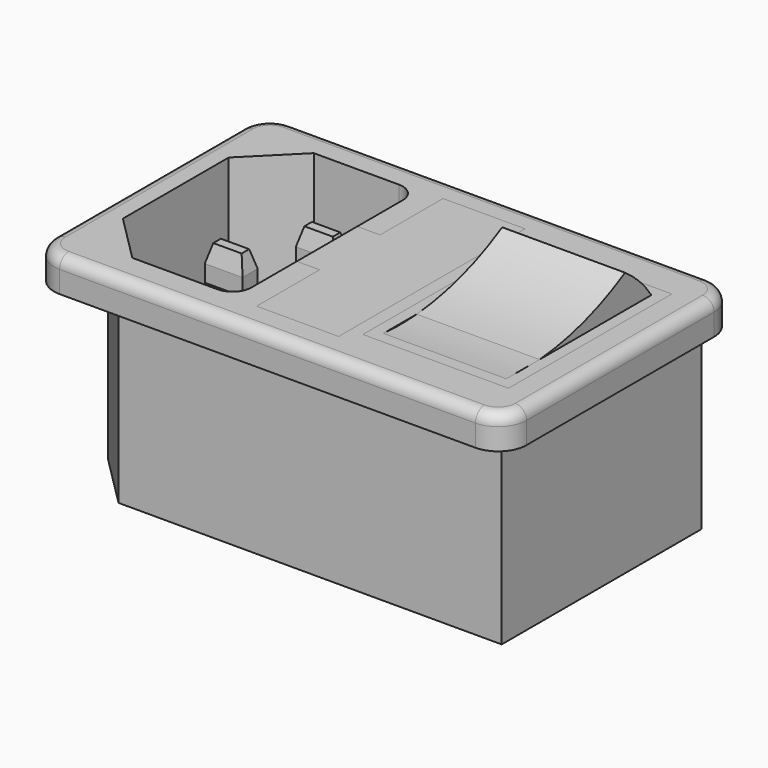
from build123d import *

# Parameters (mm, degrees)
F0_W        = 15.4
F0_H        = 21.6
F1_DEPTH    = 3.5
F0_W_2      = 4
F0_H_2      = 2
F0_W_3      = 13
F0_H_3      = 19.2
F0_W_4      = 2.418700546
F0_H_4      = 8
F2_DEPTH    = 19
F3_DEPTH    = 15
F4_C1_SIZE2 = 0.5
F4_C1_SIZE  = 1.8660254038
F4_C2_SIZE2 = 0.5
F4_C2_SIZE  = 1.8660254038
F4_C3_SIZE2 = 1.8660254038
F4_C3_SIZE  = 0.5
F4_C4_SIZE2 = 1.8660254038
F4_C4_SIZE  = 0.5
F5_SIZE2    = 1.8660254038
F5_SIZE     = 0.5
F6_SIZE2    = 1.8660254038
F6_SIZE     = 0.5
F7_DEPTH    = 3.5
F8_DEPTH    = 22
F10_DEPTH   = 25
F11_R       = 1.2
F12_START   = -14.9
F12_DEPTH   = 0.1


with BuildPart() as f1:
    # F0 (on Top) → F1 (new body)
    with BuildSketch(Plane.XY):
        with BuildLine():
            Line((21.4106866419, 15.232257545), (-22.5893133581, 15.232257545))
            ThreePointArc((-22.5893133581, 15.232257545), (-24.7106337016, 14.3535778886), (-25.5893133581, 12.232257545))
            Line((-25.5893133581, 12.232257545), (-25.5893133581, -12.567742455))
            ThreePointArc((-25.5893133581, -12.567742455), (-24.7106337016, -14.6890627986), (-22.5893133581, -15.567742455))
            Line((-22.5893133581, -15.567742455), (21.4106866419, -15.567742455))
            ThreePointArc((21.4106866419, -15.567742455), (23.5320069855, -14.6890627986), (24.4106866419, -12.567742455))
            Line((24.4106866419, -12.567742455), (24.4106866419, 12.232257545))
            ThreePointArc((24.4106866419, 12.232257545), (23.5320069855, 14.3535778886), (21.4106866419, 15.232257545))
        make_face()
        Polygon((-18.2525572471, 13.2), (-8.7555009723, 13.2), (22.2888856925, 13.2), (22.2888856925, -13.2), (-8.7555009723, -13.2), (-18.2525572471, -13.2), (-23.9555009723, -7.4970562748), (-23.9555009723, 7.4970562748), align=None, mode=Mode.SUBTRACT)
        Polygon((22.2888856925, 13.2), (-8.7555009723, 13.2), (-18.2525572471, 13.2), (-23.9555009723, 7.4970562748), (-23.9555009723, -7.4970562748), (-18.2525572471, -13.2), (-8.7555009723, -13.2), (22.2888856925, -13.2), align=None)
        with BuildLine():
            Line((-4.3368004262, 4), (-4.3368004262, 12.3322419822))
            Line((-4.3368004262, 12.3322419822), (4.3368004262, 12.3322419822))
            Line((4.3368004262, 12.3322419822), (4.3368004262, -12.3322419822))
            Line((4.3368004262, -12.3322419822), (-4.3368004262, -12.3322419822))
            Line((-4.3368004262, -12.3322419822), (-4.3368004262, -4))
            Line((-4.3368004262, -4), (-6.7555009723, -4))
            Line((-6.7555009723, -4), (-6.7555009723, -10))
            ThreePointArc((-6.7555009723, -10), (-7.3412874099, -11.4142135624), (-8.7555009723, -12))
            Line((-8.7555009723, -12), (-17.7555009723, -12))
            Line((-17.7555009723, -12), (-22.7555009723, -7))
            Line((-22.7555009723, -7), (-22.7555009723, 7))
            Line((-22.7555009723, 7), (-17.7555009723, 12))
            Line((-17.7555009723, 12), (-8.7555009723, 12))
            ThreePointArc((-8.7555009723, 12), (-7.3412874099, 11.4142135624), (-6.7555009723, 10))
            Line((-6.7555009723, 10), (-6.7555009723, 4))
            Line((-6.7555009723, 4), (-4.3368004262, 4))
        make_face(mode=Mode.SUBTRACT)
        with Locations((13.3888856925, 0)):
            Rectangle(F0_W, F0_H, mode=Mode.SUBTRACT)
    extrude(amount=F1_DEPTH)

    # F0 (on Top) → F2 (join)
    with BuildSketch(Plane.XY):
        Polygon((22.2888856925, 13.2), (-8.7555009723, 13.2), (-18.2525572471, 13.2), (-23.9555009723, 7.4970562748), (-23.9555009723, -7.4970562748), (-18.2525572471, -13.2), (-8.7555009723, -13.2), (22.2888856925, -13.2), align=None)
        with BuildLine():
            Line((-4.3368004262, 4), (-4.3368004262, 12.3322419822))
            Line((-4.3368004262, 12.3322419822), (4.3368004262, 12.3322419822))
            Line((4.3368004262, 12.3322419822), (4.3368004262, -12.3322419822))
            Line((4.3368004262, -12.3322419822), (-4.3368004262, -12.3322419822))
            Line((-4.3368004262, -12.3322419822), (-4.3368004262, -4))
            Line((-4.3368004262, -4), (-6.7555009723, -4))
            Line((-6.7555009723, -4), (-6.7555009723, -10))
            ThreePointArc((-6.7555009723, -10), (-7.3412874099, -11.4142135624), (-8.7555009723, -12))
            Line((-8.7555009723, -12), (-17.7555009723, -12))
            Line((-17.7555009723, -12), (-22.7555009723, -7))
            Line((-22.7555009723, -7), (-22.7555009723, 7))
            Line((-22.7555009723, 7), (-17.7555009723, 12))
            Line((-17.7555009723, 12), (-8.7555009723, 12))
            ThreePointArc((-8.7555009723, 12), (-7.3412874099, 11.4142135624), (-6.7555009723, 10))
            Line((-6.7555009723, 10), (-6.7555009723, 4))
            Line((-6.7555009723, 4), (-4.3368004262, 4))
        make_face(mode=Mode.SUBTRACT)
        with Locations((13.3888856925, 0)):
            Rectangle(F0_W, F0_H, mode=Mode.SUBTRACT)
        with BuildLine():
            Line((-6.7555009723, -4), (-6.7555009723, 4))
            Line((-6.7555009723, 4), (-6.7555009723, 10))
            ThreePointArc((-6.7555009723, 10), (-7.3412874099, 11.4142135624), (-8.7555009723, 12))
            Line((-8.7555009723, 12), (-17.7555009723, 12))
            Line((-17.7555009723, 12), (-22.7555009723, 7))
            Line((-22.7555009723, 7), (-22.7555009723, -7))
            Line((-22.7555009723, -7), (-17.7555009723, -12))
            Line((-17.7555009723, -12), (-8.7555009723, -12))
            ThreePointArc((-8.7555009723, -12), (-7.3412874099, -11.4142135624), (-6.7555009723, -10))
            Line((-6.7555009723, -10), (-6.7555009723, -4))
        make_face()
        with Locations((-12.8875139207, -6.9733052514)):
            Rectangle(F0_W_2, F0_H_2, mode=Mode.SUBTRACT)
        with Locations((-16.8875139207, 0)):
            Rectangle(F0_W_2, F0_H_2, mode=Mode.SUBTRACT)
        with Locations((-12.8875139207, 7.0500936662)):
            Rectangle(F0_W_2, F0_H_2, mode=Mode.SUBTRACT)
        with Locations((13.3888856925, 0)):
            Rectangle(F0_W, F0_H)
        with Locations((13.3888856925, 0)):
            Rectangle(F0_W_3, F0_H_3, mode=Mode.SUBTRACT)
        with Locations((13.3888856925, 0)):
            Rectangle(F0_W_3, F0_H_3)
        Polygon((4.3368004262, 12.3322419822), (-4.3368004262, 12.3322419822), (-4.3368004262, 4), (-4.3368004262, -4), (-4.3368004262, -12.3322419822), (4.3368004262, -12.3322419822), align=None)
        with Locations((-5.5461506993, 0)):
            Rectangle(F0_W_4, F0_H_4)
        with Locations((-12.8875139207, -6.9733052514)):
            Rectangle(F0_W_2, F0_H_2)
        with Locations((-16.8875139207, 0)):
            Rectangle(F0_W_2, F0_H_2)
        with Locations((-12.8875139207, 7.0500936662)):
            Rectangle(F0_W_2, F0_H_2)
    extrude(amount=-F2_DEPTH)

    # F0 (on Top) → F3 (cut)
    with BuildSketch(Plane.XY):
        with BuildLine():
            Line((-6.7555009723, -4), (-6.7555009723, 4))
            Line((-6.7555009723, 4), (-6.7555009723, 10))
            ThreePointArc((-6.7555009723, 10), (-7.3412874099, 11.4142135624), (-8.7555009723, 12))
            Line((-8.7555009723, 12), (-17.7555009723, 12))
            Line((-17.7555009723, 12), (-22.7555009723, 7))
            Line((-22.7555009723, 7), (-22.7555009723, -7))
            Line((-22.7555009723, -7), (-17.7555009723, -12))
            Line((-17.7555009723, -12), (-8.7555009723, -12))
            ThreePointArc((-8.7555009723, -12), (-7.3412874099, -11.4142135624), (-6.7555009723, -10))
            Line((-6.7555009723, -10), (-6.7555009723, -4))
        make_face()
        with Locations((-12.8875139207, -6.9733052514)):
            Rectangle(F0_W_2, F0_H_2, mode=Mode.SUBTRACT)
        with Locations((-16.8875139207, 0)):
            Rectangle(F0_W_2, F0_H_2, mode=Mode.SUBTRACT)
        with Locations((-12.8875139207, 7.0500936662)):
            Rectangle(F0_W_2, F0_H_2, mode=Mode.SUBTRACT)
        with Locations((13.3888856925, 0)):
            Rectangle(F0_W_3, F0_H_3)
    extrude(amount=-F3_DEPTH, mode=Mode.SUBTRACT)

    # F4: chamfer of 0.5 x 1.8660254038 on 4 edges, made by hand

    # F4_c1
    f4_c1_edges = [f1.edges().sort_by_distance(p)[0] for p in [
        (-10.8875139207, 7.0500936662, 0),
    ]]
    f4_c1_side = f1.faces().sort_by_distance((-10.8875139207, 7.0500936662, -0.01))[0]
    chamfer(f4_c1_edges, length=F4_C1_SIZE, length2=F4_C1_SIZE2, reference=f4_c1_side)

    # F4_c2
    f4_c2_edges = [f1.edges().sort_by_distance(p)[0] for p in [
        (-13.1375139207, 6.0500936662, 0),
    ]]
    f4_c2_side = f1.faces().sort_by_distance((-13.1375139207, 6.0500936662, -0.01))[0]
    chamfer(f4_c2_edges, length=F4_C2_SIZE, length2=F4_C2_SIZE2, reference=f4_c2_side)

    # F4_c3
    f4_c3_edges = [f1.edges().sort_by_distance(p)[0] for p in [
        (-14.8875139207, 7.3000936662, 0),
    ]]
    f4_c3_side = f1.faces().sort_by_distance((-14.8775139207, 7.3000936662, 0))[0]
    chamfer(f4_c3_edges, length=F4_C3_SIZE, length2=F4_C3_SIZE2, reference=f4_c3_side)

    # F4_c4
    f4_c4_edges = [f1.edges().sort_by_distance(p)[0] for p in [
        (-12.8875139207, 8.0500936662, 0),
    ]]
    f4_c4_side = f1.faces().sort_by_distance((-12.8875139207, 8.0400936662, 0))[0]
    chamfer(f4_c4_edges, length=F4_C4_SIZE, length2=F4_C4_SIZE2, reference=f4_c4_side)

    # F5
    f5_edges = [f1.edges().sort_by_distance(p)[0] for p in [
        (-16.887514, 1, 0),
        (-14.887514, 0, 0),
        (-16.887514, -1, 0),
        (-18.887514, 0, 0),
    ]]
    f5_side = f1.faces().sort_by_distance((-16.887514, 0, 0))[0]
    chamfer(f5_edges, length=F5_SIZE, length2=F5_SIZE2, reference=f5_side)

    # F6
    f6_edges = [f1.edges().sort_by_distance(p)[0] for p in [
        (-14.887514, -6.973305, 0),
        (-12.887514, -5.973305, 0),
        (-10.887514, -6.973305, 0),
        (-12.887514, -7.973305, 0),
    ]]
    f6_side = f1.faces().sort_by_distance((-12.887514, -6.973305, 0))[0]
    chamfer(f6_edges, length=F6_SIZE, length2=F6_SIZE2, reference=f6_side)


with BuildPart() as f7:
    # F7 (new, through all): a face of the model
    f7_faces = [f1.part.faces().sort_by_distance(p)[0] for p in [
        (-0.4600310991, 0, 0),
    ]]
    extrude(f7_faces, amount=F7_DEPTH)


with BuildPart() as f7b:
    # F7#2 (new, through all): a face of the model
    f7_2_faces = [f1.part.faces().sort_by_distance(p)[0] for p in [
        (13.3888856925, -10.5347227865, 0),
    ]]
    extrude(f7_2_faces, amount=F7_DEPTH)


with BuildPart() as f8:
    # F8 (new): a face of the model
    f8_faces = [f1.part.faces().sort_by_distance(p)[0] for p in [
        (13.3888856925, 0, -15),
    ]]
    extrude(f8_faces, amount=F8_DEPTH)

    # F9 (on face) → F10 (cut)
    with BuildSketch(Plane.YZ.offset(19.8888856925)):
        with BuildLine():
            ThreePointArc((-9.6, 3.5), (-7.3938840069, 3.410434439), (-5.1877680138, 3.5))
            Line((-5.1877680138, 3.5), (-9.6, 3.5))
        make_face()
        with BuildLine():
            Line((-9.6, 3.5), (-5.1877680138, 3.5))
            ThreePointArc((-5.1877680138, 3.5), (0.6561669902, 4.6282852574), (6.1150655176, 7))
            Line((6.1150655176, 7), (-9.6, 7))
            Line((-9.6, 7), (-9.6, 3.5))
        make_face()
        with BuildLine():
            ThreePointArc((6.1150655176, 7), (8.0179372576, 5.4097140483), (9.6, 3.5))
            Line((9.6, 3.5), (9.6, 7))
            Line((9.6, 7), (6.1150655176, 7))
        make_face()
    extrude(amount=-F10_DEPTH, mode=Mode.SUBTRACT)


with BuildPart() as f1_1:
    add(f1.part)

    # F11
    f11_edges = [f1_1.edges().sort_by_distance(p)[0] for p in [
        (-25.589313, -0.167742, 3.5),
        (24.410687, -0.167742, 3.5),
        (23.532007, 14.353578, 3.5),
        (-0.589313, 15.232258, 3.5),
        (-24.710634, 14.353578, 3.5),
        (-24.710634, -14.689063, 3.5),
        (-0.589313, -15.567742, 3.5),
        (23.532007, -14.689063, 3.5),
    ]]
    fillet(f11_edges, radius=F11_R)

    # F0 (on Top) → F12 (cut)
    with BuildSketch(Plane.XY.offset(F12_START)):
        with Locations((-12.8875139207, 7.0500936662)):
            Rectangle(F0_W_2, F0_H_2)
        with Locations((-16.8875139207, 0)):
            Rectangle(F0_W_2, F0_H_2)
        with Locations((-12.8875139207, -6.9733052514)):
            Rectangle(F0_W_2, F0_H_2)
    extrude(amount=-F12_DEPTH, mode=Mode.SUBTRACT)


solid = Compound([f7.part, f7b.part, f8.part, f1_1.part])
